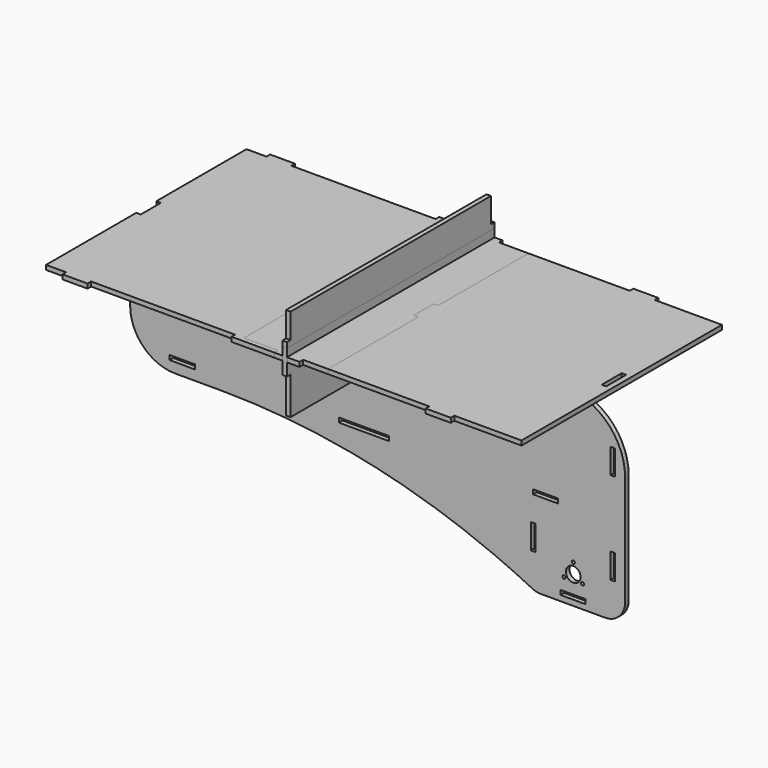
from build123d import *

# Parameters (mm, degrees)
F0_W         = 50
F0_H         = 9
F0_W_2       = 100
F0_R         = 3.07
F0_W_3       = 9
F0_H_2       = 50
F5_DEPTH     = 9
F6_R         = 40
F1_W         = 9
F1_H         = 50
F7_DEPTH     = 9
F8_DEPTH     = 9
F9_DEPTH     = 9
F10_R        = 1000
F11_T1_DEPTH = 1098.1124961061
F12_R        = 110
F13_R        = 90
F14_R        = 1400
F15_R        = 120
F16_DEPTH    = 9


# Not quite as in the source:
# - a fillet or chamfer that OpenCascade refuses, or shapes differently, is made with other operations: its cross-section is extruded or revolved along the edge and cut away or added


with BuildPart() as f5:
    # F0 (on Front) → F5 (new body)
    with BuildSketch(Plane.XZ):
        with BuildLine():
            Line((483.9999953733, -408.8390429476), (483.9999953733, -338.8390429476))
            Line((483.9999953733, -338.8390429476), (483.9999953733, -229.8390429476))
            Line((483.9999953733, -229.8390429476), (483.9999953733, -39.8390429476))
            Line((483.9999953733, -39.8390429476), (483.9999953733, -29.8390429476))
            Line((483.9999953733, -29.8390429476), (473.9999953733, -29.8390429476))
            Line((473.9999953733, -29.8390429476), (454.9999953733, -29.8390429476))
            Line((454.9999953733, -29.8390429476), (-1.0377274437, -29.8390429476))
            ThreePointArc((-1.0377274437, -29.8390429476), (-143.6076164246, -145.6589912366), (-286.1775054055, -29.8390429476))
            Line((-286.1775054055, -29.8390429476), (-494.0000046267, -29.8390429476))
            Line((-494.0000046267, -29.8390429476), (-504.0000046267, -29.8390429476))
            Line((-504.0000046267, -29.8390429476), (-504.0000046267, -39.8390429476))
            Line((-504.0000046267, -39.8390429476), (-504.0000046267, -104.8390429476))
            Line((-504.0000046267, -104.8390429476), (-504.0000046267, -258.8390429476))
            Line((-504.0000046267, -258.8390429476), (15.1211131069, -258.8390429476))
            Line((15.1211131069, -258.8390429476), (275.9999953733, -258.8390429476))
            Line((275.9999953733, -258.8390429476), (275.9999953733, -408.8390429476))
            Line((275.9999953733, -408.8390429476), (483.9999953733, -408.8390429476))
        make_face()
        with Locations((-400.0000046267, -234.3390429476)):
            Rectangle(F0_W, F0_H, mode=Mode.SUBTRACT)
        with Locations((-37.5000046267, -234.3390429476)):
            Rectangle(F0_W_2, F0_H, mode=Mode.SUBTRACT)
        Polygon((380.5047589158, -388.8390429476), (405.0242262696, -388.8390429476), (405.0242262696, -397.8390429476), (355.0242262696, -397.8390429476), (355.0242262696, -388.8390429476), align=None, mode=Mode.SUBTRACT)
        with Locations((361.9718573535, -364.0261951481)):
            Circle(F0_R, mode=Mode.SUBTRACT)
        with Locations((399.0377446354, -364.0261465598)):
            Circle(F0_R, mode=Mode.SUBTRACT)
        with BuildLine():
            ThreePointArc((395.1947869682, -353.3261708539), (390.8921756658, -363.7135793876), (380.5047589158, -368.0161708539))
            ThreePointArc((380.5047589158, -368.0161708539), (365.8147869682, -353.3261708539), (380.5047589158, -338.636170854))
            ThreePointArc((380.5047589158, -338.636170854), (390.8921756658, -342.9387623203), (395.1947869682, -353.3261708539))
        make_face(mode=Mode.SUBTRACT)
        with BuildLine():
            ThreePointArc((383.5747589158, -331.9261708539), (382.675576734, -334.0969886722), (380.5047589158, -334.9961708539))
            ThreePointArc((380.5047589158, -334.9961708539), (377.4347589158, -331.9261708539), (380.5047589158, -328.8561708539))
            ThreePointArc((380.5047589158, -328.8561708539), (382.675576734, -329.7553530357), (383.5747589158, -331.9261708539))
        make_face(mode=Mode.SUBTRACT)
        with Locations((300.5242262696, -313.8390429476)):
            Rectangle(F0_W_3, F0_H_2, mode=Mode.SUBTRACT)
        with Locations((459.5242262696, -313.8390429476)):
            Rectangle(F0_W_3, F0_H_2, mode=Mode.SUBTRACT)
        with Locations((325, -234.3390429476)):
            Rectangle(F0_W, F0_H, mode=Mode.SUBTRACT)
        with Locations((-469.5000046267, -129.8390429476)):
            Rectangle(F0_W_3, F0_H_2, mode=Mode.SUBTRACT)
        with Locations((459.4999953733, -129.8390429476)):
            Rectangle(F0_W_3, F0_H_2, mode=Mode.SUBTRACT)
    extrude(amount=F5_DEPTH)

    # F6
    f6_edges = [f5.edges().sort_by_distance(p)[0] for p in [
        (483.999995, -4.5, -408.839043),
        (275.999995, -4.5, -408.839043),
    ]]
    fillet(f6_edges, radius=F6_R)

    # F10
    f10_edges = [f5.edges().sort_by_distance(p)[0] for p in [
        (-1.037727, -4.5, -29.839043),
    ]]
    fillet(f10_edges, radius=F10_R)

    # F11: fillet of radius 500 on 1 edges, made by hand

    # F11_s2 → F11_t1 (cut)
    with BuildSketch(Plane.XZ.offset(-544.5562480531)):
        with BuildLine():
            ThreePointArc((-226.8730033326, -119.5132506089), (-358.7618430578, -54.0489361882), (-504.0000046267, -29.8390429476))
            Line((-504.0000046267, -29.8390429476), (-286.1775054055, -29.8390429476))
            ThreePointArc((-286.1775054055, -29.8390429476), (-265.1014798041, -80.3478866503), (-226.8730033326, -119.5132506089))
        make_face()
    extrude(amount=F11_T1_DEPTH, mode=Mode.SUBTRACT)

    # F12
    f12_edges = [f5.edges().sort_by_distance(p)[0] for p in [
        (-504.000005, -4.5, -29.839043),
    ]]
    fillet(f12_edges, radius=F12_R)

    # F13
    f13_edges = [f5.edges().sort_by_distance(p)[0] for p in [
        (-504.000005, -4.5, -258.839043),
    ]]
    fillet(f13_edges, radius=F13_R)

    # F14
    f14_edges = [f5.edges().sort_by_distance(p)[0] for p in [
        (275.999995, -4.5, -258.839043),
    ]]
    fillet(f14_edges, radius=F14_R)

    # F15
    f15_edges = [f5.edges().sort_by_distance(p)[0] for p in [
        (483.999995, -4.5, -29.839043),
    ]]
    fillet(f15_edges, radius=F15_R)


with BuildPart() as f7:
    # F1 (on Top) → F7 (new body)
    with BuildSketch(Plane.XY):
        Polygon((470, -250), (470, 250), (336, 250), (336, 259), (286, 259), (286, 250), (-1.5, 250), (-1.5, 259), (-101.5, 259), (-101.5, 250), (-389, 250), (-389, 259), (-439, 259), (-439, 250), (-479, 250), (-479, 25), (-470, 25), (-470, -25), (-479, -25), (-479, -250), (-439, -250), (-439, -259), (-389, -259), (-389, -250), (-101.5, -250), (-101.5, -259), (-1.5, -259), (-1.5, -250), (286, -250), (286, -259), (336, -259), (336, -250), align=None)
        with Locations((454.5, 0)):
            Rectangle(F1_W, F1_H, mode=Mode.SUBTRACT)
    extrude(amount=F7_DEPTH)


with BuildPart() as f8:
    # F3 (on face) → F8 (new body)
    with BuildSketch(Plane.XY):
        Polygon((34, -250), (84, -250), (84, -25), (75, -25), (75, 25), (84, 25), (84, 250), (25, 250), (25, 259), (-25, 259), (-25, 250), (-84, 250), (-84, 25), (-75, 25), (-75, -25), (-84, -25), (-84, -250), (-16, -250), (-16, -259), (34, -259), align=None)
    extrude(amount=F8_DEPTH)


with BuildPart() as f9:
    # F4 (on face) → F9 (new body)
    with BuildSketch(Plane.YZ):
        Polygon((250, 35.5), (250, 85.5), (25, 85.5), (-25, 85.5), (-250, 85.5), (-250, 35.5), (-259, 35.5), (-259, -14.5), (-250, -14.5), (-250, -64.5), (-25, -64.5), (-25, -73.5), (25, -73.5), (25, -64.5), (250, -64.5), (250, -14.5), (259, -14.5), (259, 35.5), align=None)
    extrude(amount=F9_DEPTH)


with BuildPart() as f16:
    # F2 (on Right) → F16 (new body)
    with BuildSketch(Plane.YZ):
        Polygon((-250, -25), (-250, -100), (-25, -100), (-25, -109), (25, -109), (25, -100), (250, -100), (250, -25), (259, -25), (259, 25), (250, 25), (-250, 25), (-259, 25), (-259, -25), align=None)
    extrude(amount=F16_DEPTH)


solid = Compound([f5.part, f7.part, f8.part, f9.part, f16.part])
